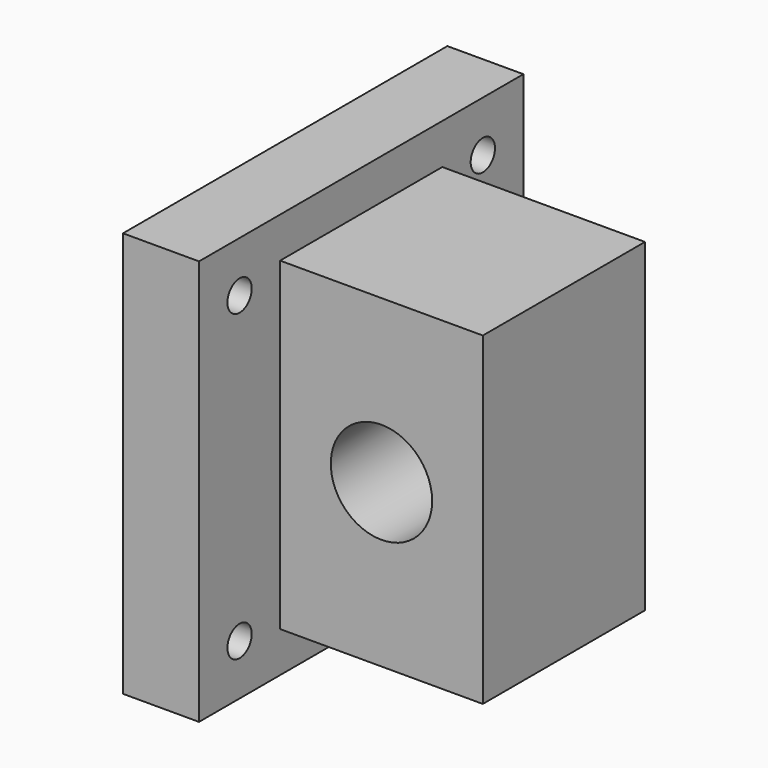
from build123d import *

# Parameters (mm, degrees)
F0_W     = 80
F0_H     = 80
F0_R     = 3
F0_W_2   = 40
F0_H_2   = 64
F1_DEPTH = 15
F2_DEPTH = 40
F3_R     = 10
F4_DEPTH = 60.001


# Not quite as in the source:
# - a feature names something its author has since deleted; it is built from what else it names


with BuildPart() as f1:
    # F0 (on Right) → F1 (new body)
    with BuildSketch(Plane.YZ):
        Rectangle(F0_W, F0_H)
        with Locations((-30, -30)):
            Circle(F0_R, mode=Mode.SUBTRACT)
        with Locations((30, -30)):
            Circle(F0_R, mode=Mode.SUBTRACT)
        with Locations((-30, 30)):
            Circle(F0_R, mode=Mode.SUBTRACT)
        Rectangle(F0_W_2, F0_H_2, mode=Mode.SUBTRACT)
        with Locations((30, 30)):
            Circle(F0_R, mode=Mode.SUBTRACT)
        Rectangle(F0_W_2, F0_H_2)
    extrude(amount=-F1_DEPTH)

    # F0 (on Right) → F2 (join)
    with BuildSketch(Plane.YZ):
        Rectangle(F0_W_2, F0_H_2)
    extrude(amount=F2_DEPTH)

    # F3 (on face) → F4 (cut, through all)
    with BuildSketch(Plane.XZ.offset(20)):
        with Locations((20, 0)):
            Circle(F3_R)
    extrude(amount=-F4_DEPTH, mode=Mode.SUBTRACT)


solid = f1.part
